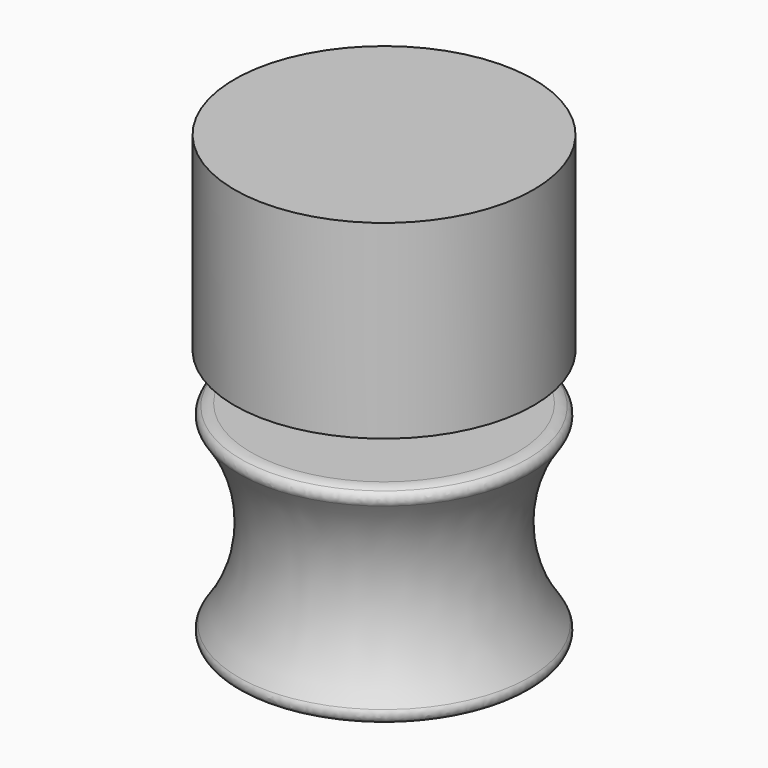
from build123d import *

# Parameters (mm, degrees)
F0_R          = 40
F1_DEPTH      = 50.8
F5_R          = 4.0613377036
F6_DEPTH      = 18.034
F5_R_2        = 11.5
F7_DEPTH      = 10
F8_DEPTH      = 20.574
F10_R         = 2.2545213031
F11_TEXT_SIZE = 2.1079521509
F12_DEPTH     = 0.508


# Not quite as in the source:
# - a fillet or chamfer that OpenCascade refuses, or shapes differently, is made with other operations: its cross-section is extruded or revolved along the edge and cut away or added
# - Text() gives the source's letters only with a copy of the font that has no kerning and outlines rounded to 1/6400 em; it was checked with that copy


with BuildPart() as f1:
    # F0 (on Top) → F1 (new body)
    with BuildSketch(Plane.XY):
        Circle(F0_R)
        Polygon((-6.7410062041, 1.1689034843), (-2.3582029901, 6.422334362), (4.3828032141, 5.2534308777), (6.7410062041, -1.1689034843), (2.3582029901, -6.422334362), (-4.3828032141, -5.2534308777), align=None, mode=Mode.SUBTRACT)
        Polygon((4.3828032141, 5.2534308777), (-2.3582029901, 6.422334362), (-6.7410062041, 1.1689034843), (-4.3828032141, -5.2534308777), (2.3582029901, -6.422334362), (6.7410062041, -1.1689034843), align=None)
    extrude(amount=F1_DEPTH)


with BuildPart() as f4:
    # F3 (on Right) → F4 (revolve)
    with BuildSketch(Plane.YZ):
        with BuildLine():
            Line((0, -12.4598681498), (-40, -12.4598681498))
            Line((-40, -12.4598681498), (-40, -14.9998681498))
            ThreePointArc((-40, -14.9998681498), (-31.2183698745, -40.3998681498), (-40, -65.7998681498))
            Line((-40, -65.7998681498), (-40, -68.3398681498))
            Line((-40, -68.3398681498), (0, -68.3398681498))
            Line((0, -68.3398681498), (0, -12.4598681498))
        make_face()
    revolve(axis=Axis((0, 0, -40.3998681498), (0, 0, -1)))

    # F5 (on face) → F6 (cut)
    with BuildSketch(Plane.XY.offset(-12.4598681498)):
        Polygon((4.3828032141, 5.2534308777), (-2.3582029901, 6.422334362), (-6.7410062041, 1.1689034843), (-4.3828032141, -5.2534308777), (2.3582029901, -6.422334362), (6.7410062041, -1.1689034843), align=None)
        Circle(F5_R, mode=Mode.SUBTRACT)
    extrude(amount=-F6_DEPTH, mode=Mode.SUBTRACT)

    # F5 (on face) → F7 (cut)
    with BuildSketch(Plane.XY.offset(-12.4598681498)):
        Circle(F5_R_2)
        Polygon((-6.7410062041, 1.1689034843), (-2.3582029901, 6.422334362), (4.3828032141, 5.2534308777), (6.7410062041, -1.1689034843), (2.3582029901, -6.422334362), (-4.3828032141, -5.2534308777), align=None, mode=Mode.SUBTRACT)
    extrude(amount=-F7_DEPTH, mode=Mode.SUBTRACT)

    # F8 (cut): a face of the model
    f8_faces = [f4.faces().sort_by_distance(p)[0] for p in [
        (0, 0, -12.4598681498),
    ]]
    extrude(f8_faces, amount=-F8_DEPTH, mode=Mode.SUBTRACT)

    # F9: fillet of radius 5.08 on 2 edges, made by hand

    # F9_s1 → F9_t2 (revolve, cut)
    with BuildSketch(Plane.YZ):
        with BuildLine():
            ThreePointArc((-35.6005909488, -12.4598681498), (-38.1405909488, -13.1404590985), (-40, -14.9998681498))
            Line((-40, -14.9998681498), (-40, -12.4598681498))
            Line((-40, -12.4598681498), (-35.6005909488, -12.4598681498))
        make_face()
    revolve(axis=Axis((0, 0, -12.4598681498), (0, 0, -1)), mode=Mode.SUBTRACT)

    # F9_s3 → F9_t4 (revolve, cut)
    with BuildSketch(Plane.YZ):
        with BuildLine():
            ThreePointArc((-40, -65.7998681498), (-38.1405909488, -67.659277201), (-35.6005909488, -68.3398681498))
            Line((-35.6005909488, -68.3398681498), (-40, -68.3398681498))
            Line((-40, -68.3398681498), (-40, -65.7998681498))
        make_face()
    revolve(axis=Axis((0, 0, -68.3398681498), (0, 0, -1)), mode=Mode.SUBTRACT)

    # F10
    f10_edges = [f4.edges().sort_by_distance(p)[0] for p in [
        (0, 40, -14.999868),
        (0, -31.21837, -40.399868),
        (0, 40, -65.799868),
    ]]
    fillet(f10_edges, radius=F10_R)

    # F11 (on face) → F12 (join)
    with BuildSketch(Plane.XY.offset(-12.4598681498)):
        with Locations((-16.4315692412, 20.8667972466)):
            Text("Evan and Steven's Motorbike", F11_TEXT_SIZE, font='Open Sans', font_style=FontStyle.BOLD, text_align=(TextAlign.LEFT, TextAlign.BOTTOM))
        with Locations((-16.4315692412, 17.9999823213)):
            Text('Designed in Massachusetts', F11_TEXT_SIZE, font='Open Sans', font_style=FontStyle.BOLD, text_align=(TextAlign.LEFT, TextAlign.BOTTOM))
    extrude(amount=F12_DEPTH)


solid = Compound([f1.part, f4.part])
